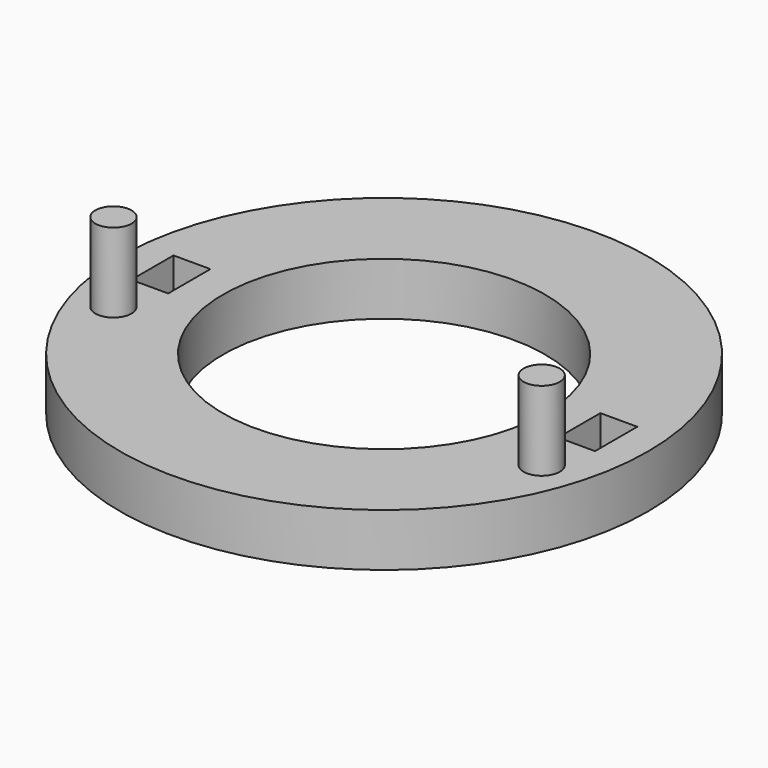
from build123d import *

# Parameters (mm, degrees)
F0_R     = 50
F0_R_2   = 3.425
F0_W     = 7
F0_H     = 10
F0_R_3   = 30.5
F1_DEPTH = 10
F2_DEPTH = 25


# Not quite as in the source:
# - a feature names something its author has since deleted; it is built from what else it names


with BuildPart() as f1:
    # F0 (on Top) → F1 (new body)
    with BuildSketch(Plane.XY):
        Circle(F0_R)
        with Locations((-40.6804330647, -13.233267504)):
            Circle(F0_R_2, mode=Mode.SUBTRACT)
        with Locations((40.4436938465, -13.233267504)):
            Circle(F0_R_2, mode=Mode.SUBTRACT)
        with Locations((-40.547645092, 0.191732496)):
            Rectangle(F0_W, F0_H, mode=Mode.SUBTRACT)
        Circle(F0_R_3, mode=Mode.SUBTRACT)
        with Locations((40.3109058738, 0.191732496)):
            Rectangle(F0_W, F0_H, mode=Mode.SUBTRACT)
        with Locations((-40.6804330647, -13.233267504)):
            Circle(F0_R_2)
        with Locations((40.4436938465, -13.233267504)):
            Circle(F0_R_2)
    extrude(amount=F1_DEPTH)

    # F0 (on Top) → F2 (join)
    with BuildSketch(Plane.XY):
        with Locations((-40.6804330647, -13.233267504)):
            Circle(F0_R_2)
        with Locations((40.4436938465, -13.233267504)):
            Circle(F0_R_2)
    extrude(amount=F2_DEPTH)


solid = f1.part
